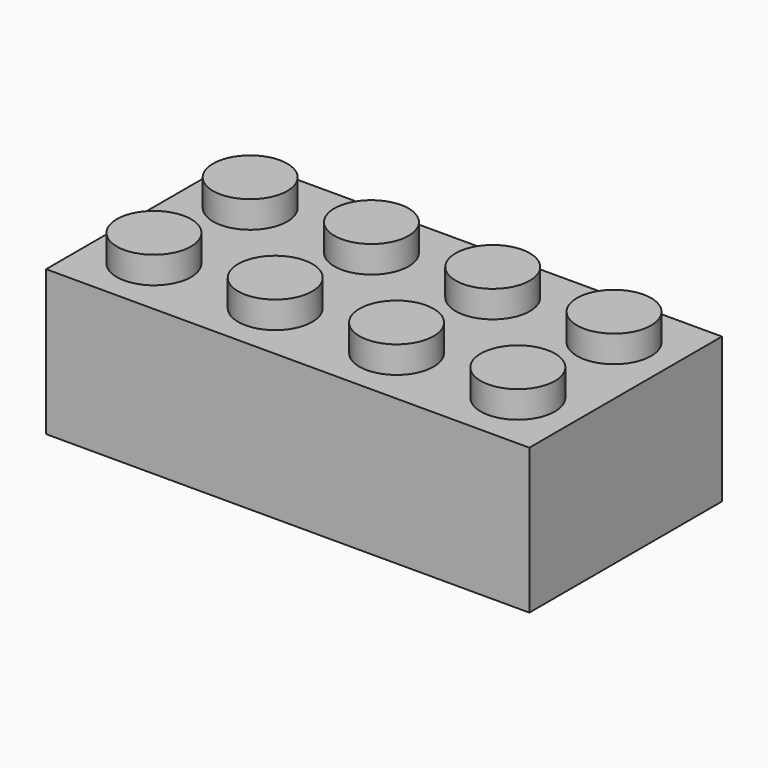
from build123d import *
from build123d import SkipClean  # not in build123d's __all__

# Parameters (mm, degrees)
F0_W         = 31.78
F0_H         = 15.83
F1_DEPTH     = 9.55
F2_R         = 2.44
F3_DEPTH     = 1.77
F4_W         = 29.34
F4_H         = 13.39
F5_DEPTH     = 8.4
F6_R         = 2.44
F7_DEPTH     = 8.4
F8_T1_DEPTH  = 17.6047426374
F8_T3_DEPTH  = 17.6047426374
F8_T5_DEPTH  = 11.4573713187
F8_T7_DEPTH  = 11.4573713187
F8_T9_DEPTH  = 13.39
F8_T14_DEPTH = 8.6771574844
F8_S15_R     = 2.44
F8_T16_DEPTH = 6
F8_T18_ANGLE = 349.8869381759
F8_T22_DEPTH = 8.6771574844
F8_S23_R     = 2.44
F8_T24_DEPTH = 6
F8_T28_DEPTH = 8.6771574844
F8_S29_R     = 2.44
F8_T30_DEPTH = 6
F8_T32_ANGLE = 349.8869381759
F8_T36_DEPTH = 8.6771574844
F8_S37_R     = 2.44
F8_T38_DEPTH = 6
F8_T42_DEPTH = 8.6771574844
F8_S43_R     = 2.44
F8_T44_DEPTH = 6
F8_T46_ANGLE = 349.8869381759
F8_T50_DEPTH = 8.6771574844
F8_S51_R     = 2.44
F8_T52_DEPTH = 6
F8_T56_DEPTH = 8.6771574844
F8_S57_R     = 2.44
F8_T58_DEPTH = 6
F8_T60_ANGLE = 349.8869381759
F8_T64_DEPTH = 8.6771574844
F8_S65_R     = 2.44
F8_T66_DEPTH = 6
F8_T70_DEPTH = 8.6771574844
F8_S71_R     = 2.44
F8_T72_DEPTH = 6
F8_T76_DEPTH = 8.6771574844
F8_S77_R     = 2.44
F8_T78_DEPTH = 6
F8_T80_ANGLE = 349.8869381759
F8_T84_DEPTH = 8.6771574844
F8_S85_R     = 2.44
F8_T86_DEPTH = 6
F8_T88_ANGLE = 349.8869381759
F8_T92_DEPTH = 8.6771574844
F8_S93_R     = 2.44
F8_T94_DEPTH = 6


# Not quite as in the source:
# - a fillet or chamfer that OpenCascade refuses, or shapes differently, is made with other operations: its cross-section is extruded or revolved along the edge and cut away or added


with BuildPart() as f1:
    # F0 (on Top) → F1 (new body)
    with BuildSketch(Plane.XY):
        with Locations((15.89, 7.915)):
            Rectangle(F0_W, F0_H)
    extrude(amount=F1_DEPTH)

    # F2 (on face) → F3 (join)
    with BuildSketch(Plane.XY.offset(9.55)):
        with Locations((27.855, 3.96)):
            Circle(F2_R)
        with Locations((27.855, 11.87)):
            Circle(F2_R)
        with Locations((19.8783333333, 3.96)):
            Circle(F2_R)
        with Locations((19.8783333333, 11.87)):
            Circle(F2_R)
        with Locations((11.9016666667, 3.96)):
            Circle(F2_R)
        with Locations((11.9016666667, 11.87)):
            Circle(F2_R)
        with Locations((3.925, 3.96)):
            Circle(F2_R)
        with Locations((3.925, 11.87)):
            Circle(F2_R)
    extrude(amount=F3_DEPTH)

    # F4 (on face) → F5 (cut)
    with BuildSketch(Plane(origin=(0, 0, 0), x_dir=(1, 0, 0), z_dir=(0, 0, -1))):
        with Locations((15.89, -7.915)):
            Rectangle(F4_W, F4_H)
    extrude(amount=-F5_DEPTH, mode=Mode.SUBTRACT)

    # F6 (on face) → F7 (join, through all)
    with BuildSketch(Plane(origin=(0, 0, 8.4), x_dir=(1, 0, 0), z_dir=(0, 0, -1))):
        with BuildLine():
            Line((15.49, -1.22), (15.49, -4.6997861657))
            ThreePointArc((15.49, -4.6997861657), (12.65, -7.915), (15.49, -11.1302138343))
            Line((15.49, -11.1302138343), (15.49, -14.61))
            Line((15.49, -14.61), (16.29, -14.61))
            Line((16.29, -14.61), (16.29, -11.1302138343))
            ThreePointArc((16.29, -11.1302138343), (19.13, -7.915), (16.29, -4.6997861657))
            Line((16.29, -4.6997861657), (16.29, -1.22))
            Line((16.29, -1.22), (15.49, -1.22))
        make_face()
        with Locations((15.89, -7.915)):
            Circle(F6_R, mode=Mode.SUBTRACT)
        with BuildLine():
            Line((24.3, -14.61), (24.3, -11.1302138343))
            ThreePointArc((24.3, -11.1302138343), (27.14, -7.915), (24.3, -4.6997861657))
            Line((24.3, -4.6997861657), (24.3, -1.22))
            Line((24.3, -1.22), (23.5, -1.22))
            Line((23.5, -1.22), (23.5, -4.6997861657))
            ThreePointArc((23.5, -4.6997861657), (20.66, -7.915), (23.5, -11.1302138343))
            Line((23.5, -11.1302138343), (23.5, -14.61))
            Line((23.5, -14.61), (24.3, -14.61))
        make_face()
        with Locations((23.9, -7.915)):
            Circle(F6_R, mode=Mode.SUBTRACT)
        with BuildLine():
            ThreePointArc((8.28, -11.1302138343), (11.12, -7.915), (8.28, -4.6997861657))
            Line((8.28, -4.6997861657), (8.28, -1.22))
            Line((8.28, -1.22), (7.48, -1.22))
            Line((7.48, -1.22), (7.48, -4.6997861657))
            ThreePointArc((7.48, -4.6997861657), (4.64, -7.915), (7.48, -11.1302138343))
            Line((7.48, -11.1302138343), (7.48, -14.61))
            Line((7.48, -14.61), (8.28, -14.61))
            Line((8.28, -14.61), (8.28, -11.1302138343))
        make_face()
        with Locations((7.88, -7.915)):
            Circle(F6_R, mode=Mode.SUBTRACT)
    extrude(amount=F7_DEPTH)

    # F8: chamfer of 2.021 on 28 edges, made by hand

    # F8_s2 → F8_t1 (join)
    with BuildSketch(Plane.YZ.offset(3.0826286813)):
        Polygon((1.22, 6.379), (3.241, 8.4), (1.22, 8.4), align=None)
        Polygon((14.61, 6.379), (12.589, 8.4), (14.61, 8.4), align=None)
    extrude(amount=F8_T1_DEPTH)

    # F8_s4 → F8_t3 (join)
    with BuildSketch(Plane.YZ.offset(11.0926286813)):
        Polygon((1.22, 6.379), (3.241, 8.4), (1.22, 8.4), align=None)
        Polygon((14.61, 6.379), (12.589, 8.4), (14.61, 8.4), align=None)
    extrude(amount=F8_T3_DEPTH)

    # F8_s6 → F8_t5 (join)
    with BuildSketch(Plane.YZ.offset(19.1026286813)):
        Polygon((1.22, 6.379), (3.241, 8.4), (1.22, 8.4), align=None)
        Polygon((14.61, 6.379), (12.589, 8.4), (14.61, 8.4), align=None)
    extrude(amount=F8_T5_DEPTH)

    # F8_s8 → F8_t7 (join)
    with BuildSketch(Plane.YZ.offset(1.22)):
        Polygon((1.22, 6.379), (3.241, 8.4), (1.22, 8.4), align=None)
        Polygon((14.61, 6.379), (12.589, 8.4), (14.61, 8.4), align=None)
    extrude(amount=F8_T7_DEPTH)

    # F8_s10 → F8_t9 (join)
    with BuildSketch(Plane.XZ.offset(-14.61)):
        Polygon((30.56, 6.379), (28.539, 8.4), (30.56, 8.4), align=None)
        Polygon((1.22, 6.379), (3.241, 8.4), (1.22, 8.4), align=None)
    extrude(amount=F8_T9_DEPTH)


with BuildPart() as f8_tool12:
    # F8_s13 → F8_t14 (new body)
    with BuildSketch(Plane.XZ.offset(-1.22)):
        Polygon((15.49, 6.379), (13.469, 8.4), (15.49, 8.4), align=None)
    extrude(amount=-F8_T14_DEPTH)

    # F8_s15 → F8_t16 (cut, symmetric)
    with BuildSketch(Plane.XY.offset(7.4)):
        with Locations((15.89, 7.915)):
            Circle(F8_S15_R)
    extrude(amount=F8_T16_DEPTH, both=True, mode=Mode.SUBTRACT)


with BuildPart() as f1_1:
    add(f1.part, clean=False)

    # F8_t11: union F8_tool12
    add(f8_tool12.part)

    # F8_s17 → F8_t18 (revolve)
    with BuildSketch(Plane(origin=(0.8183420867, 9.2485847883, 0), x_dir=(0, 0, 1), z_dir=(0.0881385962, 0.996108221, 0))):
        Polygon((6.379, 18.370542642), (8.4, 20.391542642), (8.4, 18.370542642), align=None)
    revolve(axis=Axis((15.89, 7.915, 8.4), (0, 0, -1)), revolution_arc=F8_T18_ANGLE)


with BuildPart() as f8_tool20:
    # F8_s21 → F8_t22 (new body)
    with BuildSketch(Plane.XZ.offset(-5.9328425156)):
        Polygon((15.49, 6.379), (13.469, 8.4), (15.49, 8.4), align=None)
    extrude(amount=-F8_T22_DEPTH)

    # F8_s23 → F8_t24 (cut, symmetric)
    with BuildSketch(Plane.XY.offset(7.4)):
        with Locations((15.89, 7.915)):
            Circle(F8_S23_R)
    extrude(amount=F8_T24_DEPTH, both=True, mode=Mode.SUBTRACT)


with BuildPart() as f1_2:
    add(f1_1.part, clean=False)

    # F8_t19: union F8_tool20
    add(f8_tool20.part)


with BuildPart() as f8_tool26:
    # F8_s27 → F8_t28 (new body)
    with BuildSketch(Plane.XZ.offset(-14.61)):
        Polygon((10.301, 8.4), (8.28, 6.379), (8.28, 8.4), align=None)
    extrude(amount=F8_T28_DEPTH)

    # F8_s29 → F8_t30 (cut, symmetric)
    with BuildSketch(Plane.XY.offset(7.4)):
        with Locations((7.88, 7.915)):
            Circle(F8_S29_R)
    extrude(amount=F8_T30_DEPTH, both=True, mode=Mode.SUBTRACT)


with BuildPart() as f1_3:
    add(f1_2.part, clean=False)

    # F8_t25: union F8_tool26
    add(f8_tool26.part)

    # F8_s31 → F8_t32 (revolve)
    with BuildSketch(Plane(origin=(0.7561171055, 8.5453421904, 0), x_dir=(0, 0, 1), z_dir=(-0.0881385962, -0.996108221, 0))):
        Polygon((8.4, -1.8907157922), (6.379, -3.9117157922), (8.4, -3.9117157922), align=None)
    revolve(axis=Axis((7.88, 7.915, 8.4), (0, 0, -1)), revolution_arc=F8_T32_ANGLE)


with BuildPart() as f8_tool34:
    # F8_s35 → F8_t36 (new body)
    with BuildSketch(Plane.XZ.offset(-9.8971574844)):
        Polygon((8.28, 6.379), (10.301, 8.4), (8.28, 8.4), align=None)
    extrude(amount=F8_T36_DEPTH)

    # F8_s37 → F8_t38 (cut, symmetric)
    with BuildSketch(Plane.XY.offset(7.4)):
        with Locations((7.88, 7.915)):
            Circle(F8_S37_R)
    extrude(amount=F8_T38_DEPTH, both=True, mode=Mode.SUBTRACT)


with BuildPart() as f1_4:
    add(f1_3.part, clean=False)

    # F8_t33: union F8_tool34
    add(f8_tool34.part)


with BuildPart() as f8_tool40:
    # F8_s41 → F8_t42 (new body)
    with BuildSketch(Plane.XZ.offset(-1.22)):
        Polygon((23.5, 6.379), (21.479, 8.4), (23.5, 8.4), align=None)
    extrude(amount=-F8_T42_DEPTH)

    # F8_s43 → F8_t44 (cut, symmetric)
    with BuildSketch(Plane.XY.offset(7.4)):
        with Locations((23.9, 7.915)):
            Circle(F8_S43_R)
    extrude(amount=F8_T44_DEPTH, both=True, mode=Mode.SUBTRACT)


with BuildPart() as f1_5:
    add(f1_4.part, clean=False)

    # F8_t39: union F8_tool40
    add(f8_tool40.part)

    # F8_s45 → F8_t46 (revolve)
    with BuildSketch(Plane(origin=(0.880567068, 9.9518273862, 0), x_dir=(0, 0, 1), z_dir=(0.0881385962, 0.996108221, 0))):
        Polygon((6.379, 26.3493694919), (8.4, 28.3703694919), (8.4, 26.3493694919), align=None)
    revolve(axis=Axis((23.9, 7.915, 8.4), (0, 0, -1)), revolution_arc=F8_T46_ANGLE)


with BuildPart() as f8_tool48:
    # F8_s49 → F8_t50 (new body)
    with BuildSketch(Plane.XZ.offset(-5.9328425156)):
        Polygon((23.5, 6.379), (21.479, 8.4), (23.5, 8.4), align=None)
    extrude(amount=-F8_T50_DEPTH)

    # F8_s51 → F8_t52 (cut, symmetric)
    with BuildSketch(Plane.XY.offset(7.4)):
        with Locations((23.9, 7.915)):
            Circle(F8_S51_R)
    extrude(amount=F8_T52_DEPTH, both=True, mode=Mode.SUBTRACT)


with BuildPart() as f1_6:
    add(f1_5.part, clean=False)

    # F8_t47: union F8_tool48
    add(f8_tool48.part)


with BuildPart() as f8_tool54:
    # F8_s55 → F8_t56 (new body)
    with BuildSketch(Plane.XZ.offset(-14.61)):
        Polygon((18.311, 8.4), (16.29, 6.379), (16.29, 8.4), align=None)
    extrude(amount=F8_T56_DEPTH)

    # F8_s57 → F8_t58 (cut, symmetric)
    with BuildSketch(Plane.XY.offset(7.4)):
        with Locations((15.89, 7.915)):
            Circle(F8_S57_R)
    extrude(amount=F8_T58_DEPTH, both=True, mode=Mode.SUBTRACT)


with BuildPart() as f1_7:
    add(f1_6.part, clean=False)

    # F8_t53: union F8_tool54
    add(f8_tool54.part)

    # F8_s59 → F8_t60 (revolve)
    with BuildSketch(Plane(origin=(0.8183420867, 9.2485847883, 0), x_dir=(0, 0, 1), z_dir=(-0.0881385962, -0.996108221, 0))):
        Polygon((8.4, -9.869542642), (6.379, -11.890542642), (8.4, -11.890542642), align=None)
    with SkipClean():  # cleaning this boolean's faces spoils the solid; the shape is the same uncleaned
        revolve(axis=Axis((15.89, 7.915, 8.4), (0, 0, -1)), revolution_arc=F8_T60_ANGLE)


with BuildPart() as f8_tool62:
    # F8_s63 → F8_t64 (new body)
    with BuildSketch(Plane.XZ.offset(-9.8971574844)):
        Polygon((16.29, 6.379), (18.311, 8.4), (16.29, 8.4), align=None)
    extrude(amount=F8_T64_DEPTH)

    # F8_s65 → F8_t66 (cut, symmetric)
    with BuildSketch(Plane.XY.offset(7.4)):
        with Locations((15.89, 7.915)):
            Circle(F8_S65_R)
    extrude(amount=F8_T66_DEPTH, both=True, mode=Mode.SUBTRACT)


with BuildPart() as f1_8:
    add(f1_7.part, clean=False)

    # F8_t61: union F8_tool62
    add(f8_tool62.part)


with BuildPart() as f8_tool68:
    # F8_s69 → F8_t70 (new body)
    with BuildSketch(Plane.XZ.offset(-9.8971574844)):
        Polygon((24.3, 6.379), (26.321, 8.4), (24.3, 8.4), align=None)
    extrude(amount=F8_T70_DEPTH)

    # F8_s71 → F8_t72 (cut, symmetric)
    with BuildSketch(Plane.XY.offset(7.4)):
        with Locations((23.9, 7.915)):
            Circle(F8_S71_R)
    extrude(amount=F8_T72_DEPTH, both=True, mode=Mode.SUBTRACT)


with BuildPart() as f1_9:
    add(f1_8.part, clean=False)

    # F8_t67: union F8_tool68
    add(f8_tool68.part)


with BuildPart() as f8_tool74:
    # F8_s75 → F8_t76 (new body)
    with BuildSketch(Plane.XZ.offset(-14.61)):
        Polygon((26.321, 8.4), (24.3, 6.379), (24.3, 8.4), align=None)
    extrude(amount=F8_T76_DEPTH)

    # F8_s77 → F8_t78 (cut, symmetric)
    with BuildSketch(Plane.XY.offset(7.4)):
        with Locations((23.9, 7.915)):
            Circle(F8_S77_R)
    extrude(amount=F8_T78_DEPTH, both=True, mode=Mode.SUBTRACT)


with BuildPart() as f1_10:
    add(f1_9.part, clean=False)

    # F8_t73: union F8_tool74
    add(f8_tool74.part)

    # F8_s79 → F8_t80 (revolve)
    with BuildSketch(Plane(origin=(0.880567068, 9.9518273862, 0), x_dir=(0, 0, 1), z_dir=(-0.0881385962, -0.996108221, 0))):
        Polygon((8.4, -17.8483694919), (6.379, -19.8693694919), (8.4, -19.8693694919), align=None)
    with SkipClean():  # cleaning this boolean's faces spoils the solid; the shape is the same uncleaned
        revolve(axis=Axis((23.9, 7.915, 8.4), (0, 0, -1)), revolution_arc=F8_T80_ANGLE)


with BuildPart() as f8_tool82:
    # F8_s83 → F8_t84 (new body)
    with BuildSketch(Plane.XZ.offset(-1.22)):
        Polygon((7.48, 6.379), (5.459, 8.4), (7.48, 8.4), align=None)
    extrude(amount=-F8_T84_DEPTH)

    # F8_s85 → F8_t86 (cut, symmetric)
    with BuildSketch(Plane.XY.offset(7.4)):
        with Locations((7.88, 7.915)):
            Circle(F8_S85_R)
    extrude(amount=F8_T86_DEPTH, both=True, mode=Mode.SUBTRACT)


with BuildPart() as f1_11:
    add(f1_10.part, clean=False)

    # F8_t81: union F8_tool82
    add(f8_tool82.part)

    # F8_s87 → F8_t88 (revolve)
    with BuildSketch(Plane(origin=(0.7561171055, 8.5453421904, 0), x_dir=(0, 0, 1), z_dir=(0.0881385962, 0.996108221, 0))):
        Polygon((6.379, 10.3917157922), (8.4, 12.4127157922), (8.4, 10.3917157922), align=None)
    revolve(axis=Axis((7.88, 7.915, 8.4), (0, 0, -1)), revolution_arc=F8_T88_ANGLE)


with BuildPart() as f8_tool90:
    # F8_s91 → F8_t92 (new body)
    with BuildSketch(Plane.XZ.offset(-5.9328425156)):
        Polygon((7.48, 6.379), (5.459, 8.4), (7.48, 8.4), align=None)
    extrude(amount=-F8_T92_DEPTH)

    # F8_s93 → F8_t94 (cut, symmetric)
    with BuildSketch(Plane.XY.offset(7.4)):
        with Locations((7.88, 7.915)):
            Circle(F8_S93_R)
    extrude(amount=F8_T94_DEPTH, both=True, mode=Mode.SUBTRACT)


with BuildPart() as f1_12:
    add(f1_11.part, clean=False)

    # F8_t89: union F8_tool90
    add(f8_tool90.part)


solid = f1_12.part
